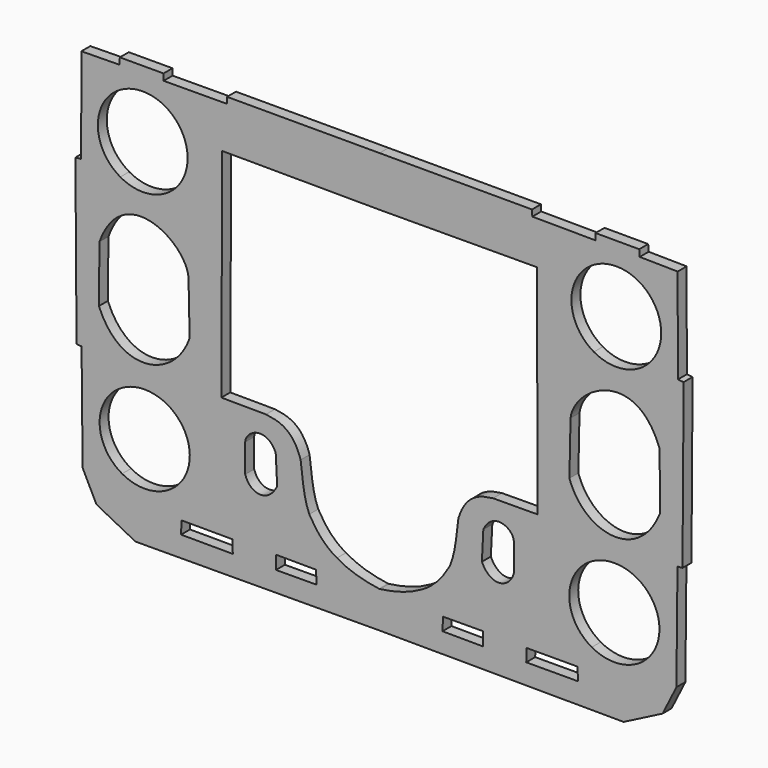
from build123d import *

# Parameters (mm, degrees)
F1_DEPTH = 4


# Not quite as in the source:
# - ends of sketch curves that miss each other by under 0.0002 mm in the source are joined


with BuildPart() as f1:
    # F0 (on Front) → F1 (new body)
    with BuildSketch(Plane.XZ):
        with BuildLine():
            Line((0, -60.8297549188), (0, -73.8967955112))
            Line((0, -73.8967955112), (87.1100496289, -74.2867405805))
            Line((87.1100496289, -74.2867405805), (101.0242826289, -67.1413325805))
            Line((101.0242826289, -67.1413325805), (105.9525546289, -57.2604655805))
            Line((105.9525546289, -57.2604655805), (106.3312226289, -19.1988875805))
            Line((106.3312226289, -19.1988875805), (108.1210446289, -19.0793755805))
            Line((108.1210446289, -19.0793755805), (108.5219496289, 39.4283344195))
            Line((108.5219496289, 39.4283344195), (106.4708796289, 39.5943924195))
            Line((106.4708796289, 39.5943924195), (106.4000046289, 73.4808784195))
            Line((106.4000046289, 73.4808784195), (92.8644466289, 73.6712574195))
            Line((92.8644466289, 73.6712574195), (92.6761516289, 76.0280454195))
            Line((92.6761516289, 76.0280454195), (77.0874396289, 76.0523674195))
            Line((77.0874396289, 76.0523674195), (77.0408646289, 73.7421304195))
            Line((77.0408646289, 73.7421304195), (54.5193526289, 73.8595534195))
            Line((54.5193526289, 73.8595534195), (54.4241656289, 76.0746004195))
            Line((54.4241656289, 76.0746004195), (0, 76.1053934693))
            Line((0, 76.1053934693), (0, 58.2839623094))
            Line((0, 58.2839623094), (56.1452326289, 58.5077654195))
            Line((56.1452326289, 58.5077654195), (56.4530356289, -19.0793755805))
            Line((56.4530356289, -19.0793755805), (40.5120526289, -19.1745575805))
            add(Edge.make_bspline(
                [(40.5120526289, -19.1745575805), (36.9506296289, -19.7234595805), (31.0349826289, -20.1211625805), (28.1548906289, -29.4563295805)],
                knots=[0, 0, 0, 0, 1, 1, 1, 1], degree=3))
            add(Edge.make_bspline(
                [(28.1548906289, -29.4563295805), (27.3785236289, -34.8808025805), (27.2311746289, -40.4625355805), (25.0629916289, -45.5390525805)],
                knots=[0, 0, 0, 0, 1, 1, 1, 1], degree=3))
            add(Edge.make_bspline(
                [(25.0629916289, -45.5390525805), (22.5362476289, -50.0321895805), (19.6081916289, -53.5319905805), (15.1727896289, -56.0456005805)],
                knots=[0, 0, 0, 0, 1, 1, 1, 1], degree=3))
            add(Edge.make_bspline(
                [(15.1727896289, -56.0456005805), (10.4594036477, -58.820394717), (5.445743624, -60.1029114405), (0.1550796733, -60.8297549188)],
                knots=[0, 0, 0, 0, 0.9984504356, 0.9984504356, 0.9984504356, 0.9984504356], degree=3))
            Line((0.1550796733, -60.8297549188), (0, -60.8297549188))
        make_face()
        Polygon((22.4935926289, -66.8113025805), (22.6353336289, -62.1665075805), (36.8552756289, -62.0956475805), (36.9483786289, -66.8821775805), align=None, mode=Mode.SUBTRACT)
        with BuildLine():
            Line((36.5252426289, -40.4245775805), (37.0456556289, -30.1386355805))
            add(Edge.make_bspline(
                [(47.9388526289, -30.2581405805), (47.5903856289, -26.1010925805), (40.1854096289, -22.9941275805), (37.0456556289, -30.1386355805)],
                knots=[0, 0, 0, 0, 1, 1, 1, 1], degree=3))
            Line((47.9388526289, -30.2581405805), (47.9166236289, -40.4245775805))
            add(Edge.make_bspline(
                [(36.5252426289, -40.4245775805), (39.5748886289, -47.0515105805), (46.1937256289, -46.0800805805), (47.9166236289, -40.4245775805)],
                knots=[0, 0, 0, 0, 1, 1, 1, 1], degree=3))
        make_face(mode=Mode.SUBTRACT)
        Polygon((52.3508896289, -66.8578555805), (52.5391806289, -62.3061655805), (70.6729776289, -62.2595755805), (70.8147186289, -66.8091795805), align=None, mode=Mode.SUBTRACT)
        with BuildLine():
            add(Edge.make_bspline(
                [(91.8478096289, -27.5109605805), (96.8262026289, -30.2957185805), (99.8930176289, -35.4421625805), (99.8930176289, -41.0116775805)],
                knots=[0, 0, 0, 0, 1, 1, 1, 1], degree=3))
            add(Edge.make_bspline(
                [(99.8930176289, -41.0116775805), (99.8930176289, -46.5811925805), (96.8262026289, -51.7276365805), (91.8478096289, -54.5123945805)],
                knots=[0, 0, 0, 0, 1, 1, 1, 1], degree=3))
            add(Edge.make_bspline(
                [(91.8478096289, -54.5123945805), (86.8694176289, -57.2971515805), (80.7357866289, -57.2971515805), (75.7573936289, -54.5123945805)],
                knots=[0, 0, 0, 0, 1, 1, 1, 1], degree=3))
            add(Edge.make_bspline(
                [(75.7573936289, -54.5123945805), (70.7790016289, -51.7276365805), (67.7121856289, -46.5811925805), (67.7121856289, -41.0116775805)],
                knots=[0, 0, 0, 0, 1, 1, 1, 1], degree=3))
            add(Edge.make_bspline(
                [(67.7121856289, -41.0116775805), (67.7121856289, -35.4421625805), (70.7790016289, -30.2957185805), (75.7573936289, -27.5109605805)],
                knots=[0, 0, 0, 0, 1, 1, 1, 1], degree=3))
            add(Edge.make_bspline(
                [(75.7573936289, -27.5109605805), (80.7357866289, -24.7262035805), (86.8694176289, -24.7262035805), (91.8478096289, -27.5109605805)],
                knots=[0, 0, 0, 0, 1, 1, 1, 1], degree=3))
        make_face(mode=Mode.SUBTRACT)
        with BuildLine():
            add(Edge.make_bspline(
                [(68.1673266289, 15.0146874195), (69.4436526289, 25.8273554195), (91.6549896289, 38.5868954195), (99.9389866289, 15.7162674195)],
                knots=[0, 0, 0, 0, 1, 1, 1, 1], degree=3))
            Line((99.9389866289, 15.7162674195), (100.1394466289, -4.5293975805))
            add(Edge.make_bspline(
                [(100.1394466289, -4.5293975805), (92.4962496289, -23.3266025805), (72.9593576289, -19.3084625805), (67.7664206289, -4.0282625805)],
                knots=[0, 0, 0, 0, 1, 1, 1, 1], degree=3))
            Line((67.7664206289, -4.0282625805), (68.1673266289, 15.0146874195))
        make_face(mode=Mode.SUBTRACT)
        with BuildLine():
            add(Edge.make_bspline(
                [(92.5110916289, 65.8933484195), (97.4657886289, 63.0685594195), (100.5180086289, 57.8481334195), (100.5180086289, 52.1985554195)],
                knots=[0, 0, 0, 0, 1, 1, 1, 1], degree=3))
            add(Edge.make_bspline(
                [(100.5180086289, 52.1985554195), (100.5180086289, 46.5489774195), (97.4657886289, 41.3285514195), (92.5110916289, 38.5037624195)],
                knots=[0, 0, 0, 0, 1, 1, 1, 1], degree=3))
            add(Edge.make_bspline(
                [(92.5110916289, 38.5037624195), (87.5563936289, 35.6789734195), (81.4519556289, 35.6789734195), (76.4972576289, 38.5037624195)],
                knots=[0, 0, 0, 0, 1, 1, 1, 1], degree=3))
            add(Edge.make_bspline(
                [(76.4972576289, 38.5037624195), (71.5425606289, 41.3285514195), (68.4903406289, 46.5489774195), (68.4903406289, 52.1985554195)],
                knots=[0, 0, 0, 0, 1, 1, 1, 1], degree=3))
            add(Edge.make_bspline(
                [(68.4903406289, 52.1985554195), (68.4903406289, 57.8481334195), (71.5425606289, 63.0685594195), (76.4972576289, 65.8933484195)],
                knots=[0, 0, 0, 0, 1, 1, 1, 1], degree=3))
            add(Edge.make_bspline(
                [(76.4972576289, 65.8933484195), (81.4519556289, 68.7181374195), (87.5563936289, 68.7181374195), (92.5110916289, 65.8933484195)],
                knots=[0, 0, 0, 0, 1, 1, 1, 1], degree=3))
        make_face(mode=Mode.SUBTRACT)
    extrude(amount=F1_DEPTH)

    # F2: F1 across plane


with BuildPart() as f1_1:
    add(f1.part)
    add(f1.part.mirror(Plane.YZ))


solid = f1_1.part
